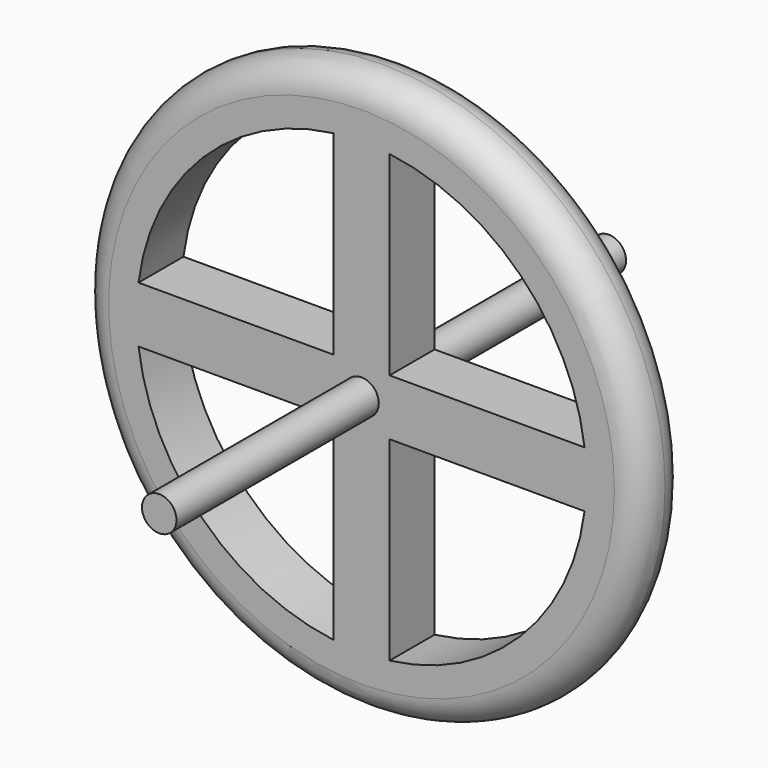
from build123d import *

# Parameters (mm, degrees)
F0_R     = 63.5
F0_R_2   = 3.81
F1_DEPTH = 6.35
F2_R     = 6.34999
F3_R     = 3.9002189419
F4_DEPTH = 63.5


# Not quite as in the source:
# - a fillet or chamfer is up to 0.001 mm smaller than in the source, because OpenCascade refuses the exact size


with BuildPart() as f1:
    # F0 (on Front) → F1 (new body, symmetric)
    with BuildSketch(Plane.XZ):
        Circle(F0_R)
        with BuildLine():
            ThreePointArc((-6.35, -50.4015624758), (-35.9210244843, -35.9210244843), (-50.4015624758, -6.35))
            Line((-50.4015624758, -6.35), (-6.35, -6.35))
            Line((-6.35, -6.35), (-6.35, -50.4015624758))
        make_face(mode=Mode.SUBTRACT)
        with BuildLine():
            Line((6.35, -50.4015624758), (6.35, -6.35))
            Line((6.35, -6.35), (50.4015624758, -6.35))
            ThreePointArc((50.4015624758, -6.35), (35.9210244843, -35.9210244843), (6.35, -50.4015624758))
        make_face(mode=Mode.SUBTRACT)
        with BuildLine():
            Line((-6.3499999233, 50.4015624854), (-6.3499999233, 6.35))
            Line((-6.3499999233, 6.35), (-50.4015624758, 6.35))
            ThreePointArc((-50.4015624758, 6.35), (-35.9210244569, 35.9210245116), (-6.3499999233, 50.4015624854))
        make_face(mode=Mode.SUBTRACT)
        Circle(F0_R_2, mode=Mode.SUBTRACT)
        with BuildLine():
            Line((50.4015624854, 6.3499999233), (6.35, 6.3499999233))
            Line((6.35, 6.3499999233), (6.35, 50.4015624758))
            ThreePointArc((6.35, 50.4015624758), (35.9210245116, 35.9210244569), (50.4015624854, 6.3499999233))
        make_face(mode=Mode.SUBTRACT)
    extrude(amount=F1_DEPTH, both=True)

    # F2 (radius 6.35 in the source; OpenCascade refuses exactly that, so slightly less here)
    f2_edges = [f1.edges().sort_by_distance(p)[0] for p in [
        (-63.5, 6.35, 0),
        (63.5, 0, 0),
        (-63.5, -6.35, 0),
    ]]
    fillet(f2_edges, radius=F2_R)

    # F3 (on Front) → F4 (join, symmetric)
    with BuildSketch(Plane.XZ):
        with Locations((4.138e-07, 0)):
            Circle(F3_R)
    extrude(amount=F4_DEPTH, both=True)


solid = f1.part
